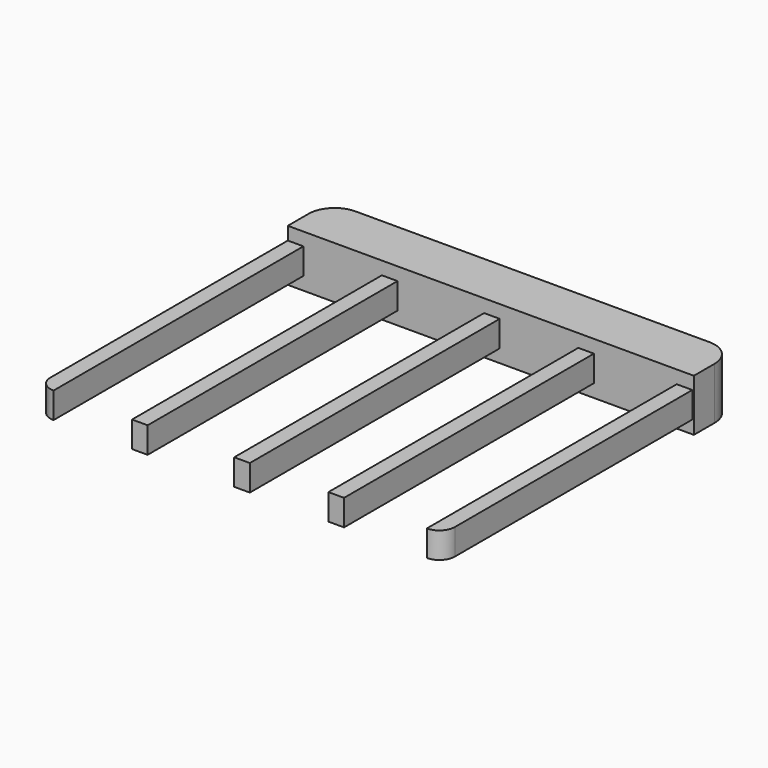
from build123d import *

# Parameters (mm, degrees)
F1_DEPTH = 6.35
F0_W     = 3.81
F0_H     = 76.2000009209
F0_H_2   = 76.2
F2_DEPTH = 3.175


# Not quite as in the source:
# - ends of sketch curves that miss each other by under 0.0002 mm in the source are joined


with BuildPart() as f1:
    # F0 (on Top) → F1 (new body, symmetric)
    with BuildSketch(Plane.XY):
        with BuildLine():
            Line((-49.2071506187, 28.1480993807), (-49.2071506187, 21.7980993807))
            Line((-49.2071506187, 21.7980993807), (-45.3971506187, 21.7980993807))
            Line((-45.3971506187, 21.7980993807), (-26.2557423981, 21.7980993807))
            Line((-26.2557423981, 21.7980993807), (-22.4457423981, 21.7980993807))
            Line((-22.4457423981, 21.7980993807), (-1.3203332201, 21.7980993807))
            Line((-1.3203332201, 21.7980993807), (2.4896667799, 21.7980993807))
            Line((2.4896667799, 21.7980993807), (21.6630548239, 21.7980993807))
            Line((21.6630548239, 21.7980993807), (25.4730548239, 21.7980993807))
            Line((25.4730548239, 21.7980993807), (45.6722128358, 21.7980993807))
            Line((45.6722128358, 21.7980993807), (49.4822128358, 21.7980993807))
            Line((49.4822128358, 21.7980993807), (49.8528493813, 21.7980993807))
            Line((49.8528493813, 21.7980993807), (49.8528493813, 28.1480993807))
            ThreePointArc((49.8528493813, 28.1480993807), (47.9929774418, 32.6382274413), (43.5028493813, 34.4980993807))
            Line((43.5028493813, 34.4980993807), (-42.8571506187, 34.4980993807))
            ThreePointArc((-42.8571506187, 34.4980993807), (-47.3472786793, 32.6382274413), (-49.2071506187, 28.1480993807))
        make_face()
    extrude(amount=F1_DEPTH, both=True)

    # F0 (on Top) → F2 (join, symmetric)
    with BuildSketch(Plane.XY):
        with BuildLine():
            Line((-49.2071506187, 28.1480993807), (-49.2071506187, 21.7980993807))
            Line((-49.2071506187, 21.7980993807), (-45.3971506187, 21.7980993807))
            Line((-45.3971506187, 21.7980993807), (-26.2557423981, 21.7980993807))
            Line((-26.2557423981, 21.7980993807), (-22.4457423981, 21.7980993807))
            Line((-22.4457423981, 21.7980993807), (-1.3203332201, 21.7980993807))
            Line((-1.3203332201, 21.7980993807), (2.4896667799, 21.7980993807))
            Line((2.4896667799, 21.7980993807), (21.6630548239, 21.7980993807))
            Line((21.6630548239, 21.7980993807), (25.4730548239, 21.7980993807))
            Line((25.4730548239, 21.7980993807), (45.6722128358, 21.7980993807))
            Line((45.6722128358, 21.7980993807), (49.4822128358, 21.7980993807))
            Line((49.4822128358, 21.7980993807), (49.8528493813, 21.7980993807))
            Line((49.8528493813, 21.7980993807), (49.8528493813, 28.1480993807))
            ThreePointArc((49.8528493813, 28.1480993807), (47.9929774418, 32.6382274413), (43.5028493813, 34.4980993807))
            Line((43.5028493813, 34.4980993807), (-42.8571506187, 34.4980993807))
            ThreePointArc((-42.8571506187, 34.4980993807), (-47.3472786793, 32.6382274413), (-49.2071506187, 28.1480993807))
        make_face()
        with BuildLine():
            Line((-45.3971506187, 21.7980993807), (-49.2071506187, 21.7980993807))
            Line((-49.2071506187, 21.7980993807), (-49.2071506187, -50.5919006193))
            ThreePointArc((-49.2071506187, -50.5919006193), (-48.0912274551, -53.2859774556), (-45.3971506187, -54.4019006193))
            Line((-45.3971506187, -54.4019006193), (-45.3971506187, 21.7980993807))
        make_face()
        with Locations((-24.3507423981, -16.3019010797)):
            Rectangle(F0_W, F0_H)
        with Locations((0.5846667799, -16.3019006193)):
            Rectangle(F0_W, F0_H_2)
        with Locations((23.5680548239, -16.3019006193)):
            Rectangle(F0_W, F0_H_2)
        with BuildLine():
            Line((49.4822128358, -50.5919006193), (49.4822128358, 21.7980993807))
            Line((49.4822128358, 21.7980993807), (45.6722128358, 21.7980993807))
            Line((45.6722128358, 21.7980993807), (45.6722128358, -54.4019006193))
            ThreePointArc((45.6722128358, -54.4019006193), (48.3662896722, -53.2859774556), (49.4822128358, -50.5919006193))
        make_face()
    extrude(amount=F2_DEPTH, both=True)


solid = f1.part
